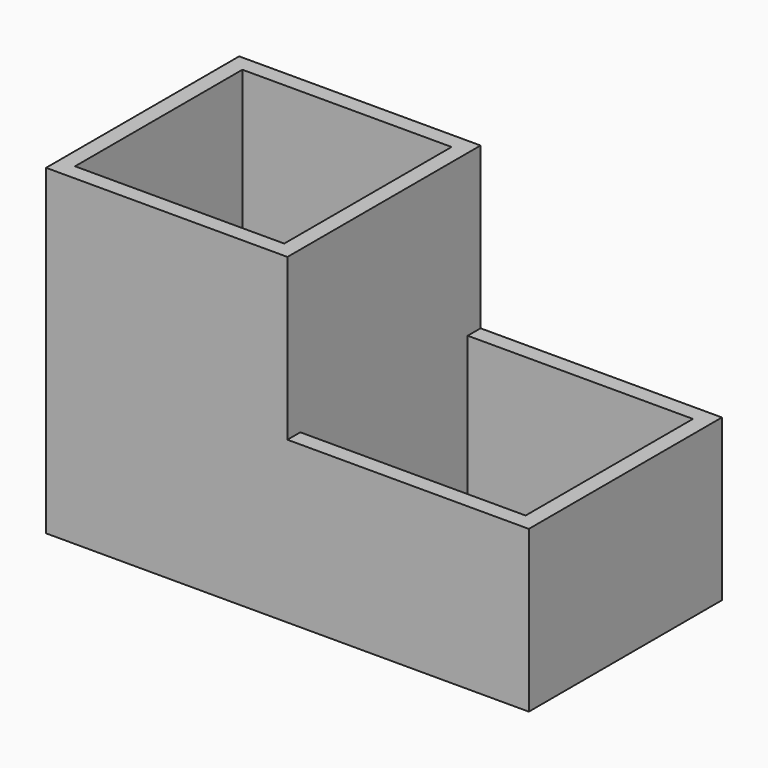
from build123d import *

# Parameters (mm, degrees)
F0_W     = 38.1
F0_H     = 38.1
F1_DEPTH = 50.8
F2_T     = -2.54
F3_DEPTH = 25.4
F4_T     = -2.54


# Not quite as in the source:
# - a shell that OpenCascade refuses in one call is made with other operations: the cavity is built on its own and cut out


with BuildPart() as f1:
    # F0 (on Top) → F1 (new body)
    with BuildSketch(Plane.XY):
        Rectangle(F0_W, F0_H)
    extrude(amount=F1_DEPTH)

    # F2
    f2_openings = [f1.faces().sort_by_distance(p)[0] for p in [
        (0, 0, 50.8),
    ]]
    offset(amount=F2_T, openings=f2_openings)

    # F0 (on Top) → F3 (join)
    with BuildSketch(Plane.XY):
        with Locations((38.1, 0)):
            Rectangle(F0_W, F0_H)
    extrude(amount=F3_DEPTH)

    # F4: a shell. OpenCascade refuses it in one call, so the cavity is built on its own and cut out:
    # the body offset inwards by the wall thickness, plus a prism from it out through each open face.
    f4_core = offset(f1.part, amount=F4_T, kind=Kind.INTERSECTION, mode=Mode.PRIVATE)
    f4_exits = [f4_core.faces().sort_by_distance(p)[0] for p in [
        (36.83, 0, 22.86),
    ]]
    add(f4_core, mode=Mode.SUBTRACT)
    extrude(f4_exits, amount=-F4_T, mode=Mode.SUBTRACT)


solid = f1.part
